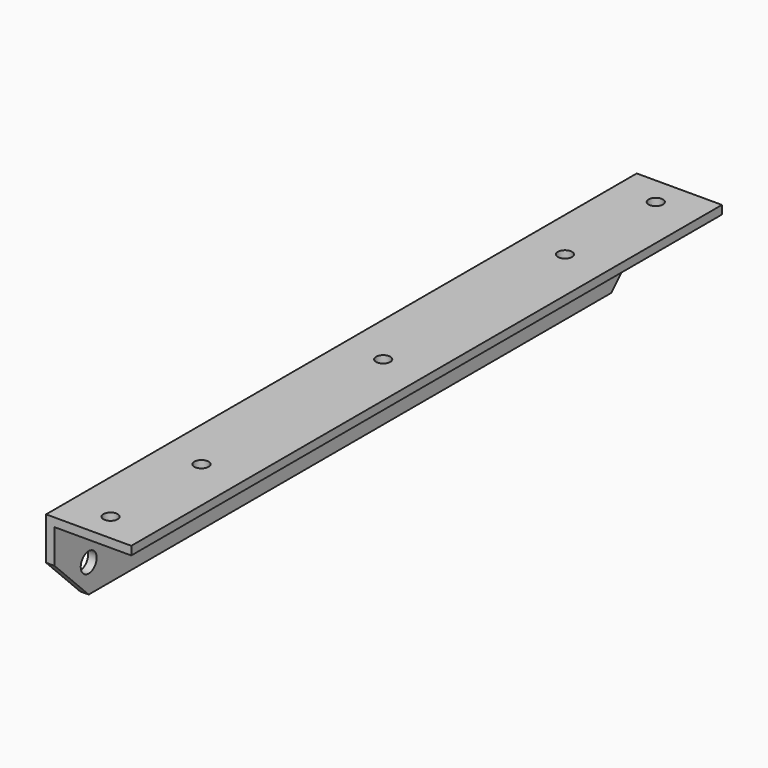
from build123d import *

# Parameters (mm, degrees)
F1_DEPTH = 130
F3_D     = 7
F5_D     = 5
F7_DEPTH = 25


# Not quite as in the source:
# - a feature names something its author has since deleted; it is built from what else it names


with BuildPart() as f1:
    # F0 (on Front) → F1 (new body, symmetric)
    with BuildSketch(Plane.XZ):
        Polygon((0, 30), (0, 0), (3, 0), (3, 27), (30, 27), (30, 30), align=None)
    extrude(amount=F1_DEPTH, both=True)

    # F3 (through all)
    with Locations(Plane(origin=(0, 0, 0), x_dir=(0, -1, 0), z_dir=(-1, 0, 0))):
        with Locations((-115, 10), (-30, 10), (30, 10), (115, 10)):
            Hole(F3_D / 2)

    # F5 (through all)
    with Locations(Plane.XY.offset(30)):
        with Locations((14.7187495604, -120), (14.7187495604, -80), (14.7187495604, 0), (14.7187495604, 80), (14.7187495604, 120)):
            Hole(F5_D / 2)

    # F6 (on face) → F7 (cut)
    with BuildSketch(Plane.YZ.offset(3)):
        Polygon((-130, 15), (-130, 0), (-115, 0), align=None)
        Polygon((130, 15), (115, 0), (130, 0), align=None)
    extrude(amount=-F7_DEPTH, mode=Mode.SUBTRACT)


solid = f1.part
